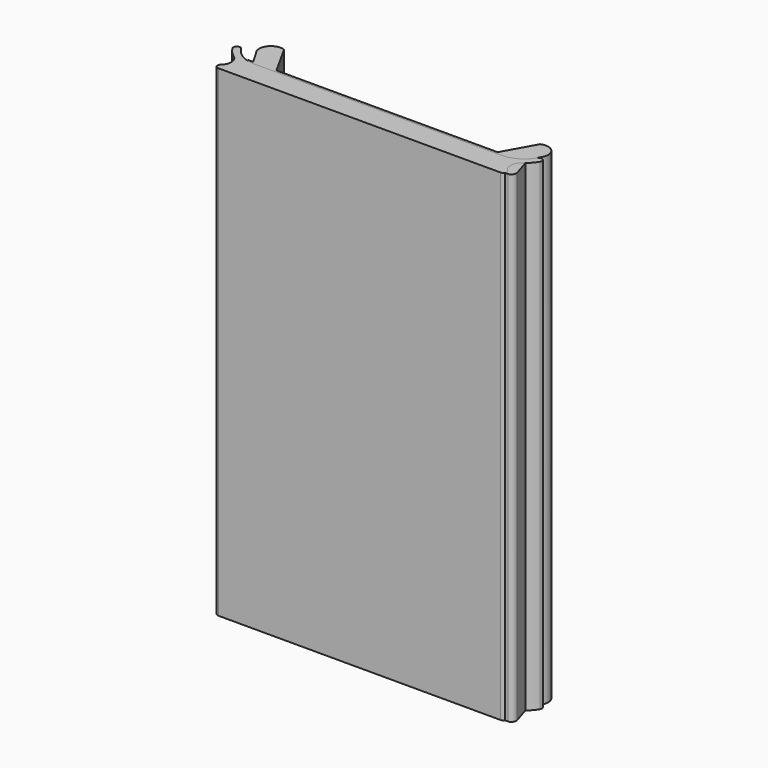
from build123d import *

# Parameters (mm, degrees)
F1_DEPTH = 250
F2_SCALE = 0.1
F4_DEPTH = 25


# Not quite as in the source:
# - ends of sketch curves that miss each other by under 0.0002 mm in the source are joined


with BuildPart() as f1:
    # F0 (on Top) → F1 (new body)
    with BuildSketch(Plane.XY):
        with BuildLine():
            Line((-53.633557, 1.195441), (-62.6724906028, 17.4106930814))
            ThreePointArc((-62.6724906028, 17.4106930814), (-69.142266545, 16.1210302987), (-70.6766850708, 9.7048951206))
            Line((-70.6766850708, 9.7048951206), (-65.684308, 1.195441))
            Line((-65.684308, 1.195441), (-68.17694, 1.195441))
            Line((-68.17694, 1.195441), (-71.1491983328, -8.1931208927))
            ThreePointArc((-71.1491983328, -8.1931208927), (-70.3707522269, -10.3869306581), (-68.1769443193, -11.165382))
            Line((-68.1769443193, -11.165382), (76.3786361624, -11.165382))
            ThreePointArc((76.3786361624, -11.165382), (78.0948325124, -10.1247630324), (78.6397955471, -8.1931230456))
            Line((78.6397955471, -8.1931230456), (75.667537, 1.195441))
            Line((75.667537, 1.195441), (73.174905, 1.195441))
            Line((73.174905, 1.195441), (77.7065557459, 8.9645952796))
            ThreePointArc((77.7065557459, 8.9645952796), (77.0978016072, 16.0125981458), (70.1630878027, 17.41069344))
            Line((70.1630878027, 17.41069344), (61.124154, 1.195441))
            Line((61.124154, 1.195441), (-53.633557, 1.195441))
        make_face()
    extrude(amount=F1_DEPTH)


with BuildPart() as f1_1:
    # F2: moved
    add(f1.part.scale(F2_SCALE))


with BuildPart() as f4:
    # F3 (on Top) → F4 (new body)
    with BuildSketch(Plane.XY):
        with BuildLine():
            ThreePointArc((7.9742238776, 0.5335820896), (7.9164179104, 0.7742238776), (7.6757761224, 0.7164179104))
            ThreePointArc((7.6757761224, 0.7164179104), (7.1297309804, 0.1913034855), (6.3967143143, 0))
            Line((6.3967143143, 0), (0, 0))
            Line((0, 0), (-6.3967143143, 0))
            ThreePointArc((-6.3967143143, 0), (-7.1297309804, 0.1913034855), (-7.6757761224, 0.7164179104))
            ThreePointArc((-7.6757761224, 0.7164179104), (-7.9164179104, 0.7742238776), (-7.9742238776, 0.5335820896))
            ThreePointArc((-7.9742238776, 0.5335820896), (-7.7533706188, 0.2422306764), (-7.4795347057, 0))
            ThreePointArc((-7.4795347057, 0), (-7.2437138511, -0.4367609962), (-7.4396680049, -0.8928022366))
            ThreePointArc((-7.4396680049, -0.8928022366), (-7.4889506154, -1.0861980041), (-7.325, -1.2))
            Line((-7.325, -1.2), (0, -1.2))
            Line((0, -1.2), (7.325, -1.2))
            ThreePointArc((7.325, -1.2), (7.4889506154, -1.0861980041), (7.4396680049, -0.8928022366))
            ThreePointArc((7.4396680049, -0.8928022366), (7.2437138511, -0.4367609962), (7.4795347057, 0))
            ThreePointArc((7.4795347057, 0), (7.7533706188, 0.2422306764), (7.9742238776, 0.5335820896))
        make_face()
    extrude(amount=F4_DEPTH)


solid = Compound([f1_1.part, f4.part])
